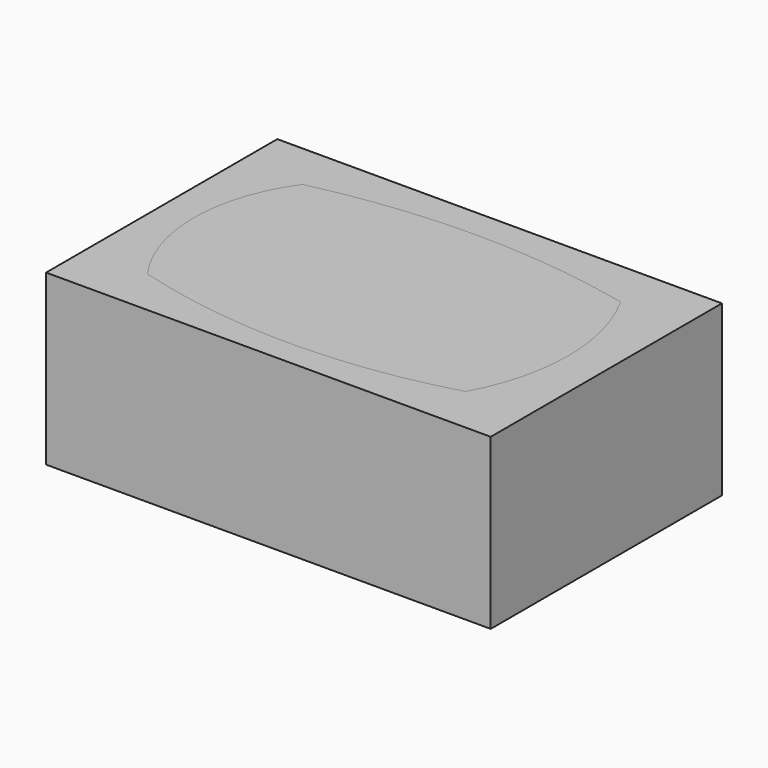
from build123d import *

# Parameters (mm, degrees)
F0_W     = 133.5640400648
F0_H     = 86.8166312575
F2_DEPTH = 50.8


# Not quite as in the source:
# - a feature of the source that left no trace in its solid (it failed there, or was rolled back) is left out


with BuildPart() as f2:
    # F0 (on Top) → F2 (new body)
    with BuildSketch(Plane.XY):
        Rectangle(F0_W, F0_H)
        with BuildLine():
            ThreePointArc((-47.8078350425, 29.1058067232), (0, 34.5567017881), (47.8078350425, 29.1058067232))
            ThreePointArc((47.8078350425, 29.1058067232), (55.2757817597, 0), (47.8078350425, -29.1058067232))
            ThreePointArc((47.8078350425, -29.1058067232), (0, -35.794125029), (-47.8078350425, -29.1058067232))
            ThreePointArc((-47.8078350425, -29.1058067232), (-57.1202847567, 0), (-47.8078350425, 29.1058067232))
        make_face(mode=Mode.SUBTRACT)
    extrude(amount=F2_DEPTH)


with BuildPart() as f2b:
    # F1 (on face) → F2, piece 2 (new body)
    with BuildSketch(Plane.XY):
        with BuildLine():
            ThreePointArc((47.8078350425, 29.1058067232), (0, 34.5567017881), (-47.8078350425, 29.1058067232))
            ThreePointArc((-47.8078350425, 29.1058067232), (-57.1202847567, 0), (-47.8078350425, -29.1058067232))
            ThreePointArc((-47.8078350425, -29.1058067232), (0, -35.794125029), (47.8078350425, -29.1058067232))
            ThreePointArc((47.8078350425, -29.1058067232), (55.2757817597, 0), (47.8078350425, 29.1058067232))
        make_face()
    extrude(amount=F2_DEPTH)


solid = Compound([f2.part, f2b.part])
